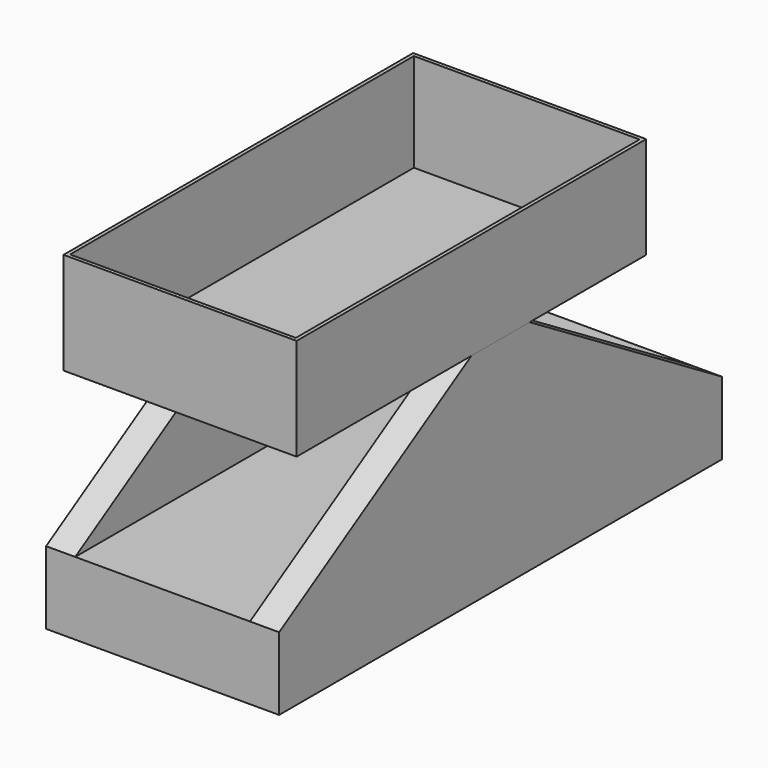
from build123d import *

# Parameters (mm, degrees)
F1_W      = 160
F1_H      = 380
F2_DEPTH  = 50
F3_W      = 20
F3_H      = 100
F5_W      = 20
F5_H      = 50
F10_DEPTH = 70
F11_T     = -2.5
F13_DEPTH = 20
F15_DEPTH = 20


# Not quite as in the source:
# - a feature of the source that left no trace in its solid (it failed there, or was rolled back) is left out
# - a pattern or mirror of a feature is missing from the dataset's text; its kind, count and spacing are read off the source's solid


with BuildPart() as f2:
    # F1 (on offset) → F2 (new body)
    with BuildSketch(Plane.XY.offset(275)):
        Rectangle(F1_W, F1_H)
    extrude(amount=-F2_DEPTH)

    # F3 (on face) → F7 section 0
    with BuildSketch(Plane.XY.offset(275)):
        with Locations((-70, -140)):
            Rectangle(F3_W, F3_H)
    # F5 (on offset) → F7 section 1
    with BuildSketch(Plane.XY.offset(375)):
        with Locations((-70, 0)):
            Rectangle(F5_W, F5_H)
    f7 = loft()

    # F7_copies: F7 across plane
    add(f7.mirror(Plane(origin=(0, 0, 0), x_dir=(0, 0, 1), z_dir=(1, 0, 0))))

    # F12 (on face) → F13 (join)
    with BuildSketch(Plane.YZ.offset(80)):
        Polygon((25, 375), (-90, 275), (190, 275), align=None)
    extrude(amount=-F13_DEPTH)

    # F14 (on face) → F15 (join)
    with BuildSketch(Plane(origin=(-80, 0, 0), x_dir=(0, -1, 0), z_dir=(-1, 0, 0))):
        Polygon((-190, 275), (90, 275), (-25, 375), align=None)
    extrude(amount=-F15_DEPTH)


with BuildPart() as f10:
    # F9 (on face) → F10 (new body)
    with BuildSketch(Plane.XY.offset(375)):
        Polygon((-80, -175), (80, -175), (80, 125), (-80, 125), (-80, -25), align=None)
    extrude(amount=F10_DEPTH)

    # F11
    f11_openings = [f10.faces().sort_by_distance(p)[0] for p in [
        (0, -25, 445),
    ]]
    offset(amount=F11_T, openings=f11_openings)


solid = Compound([f2.part, f10.part])
